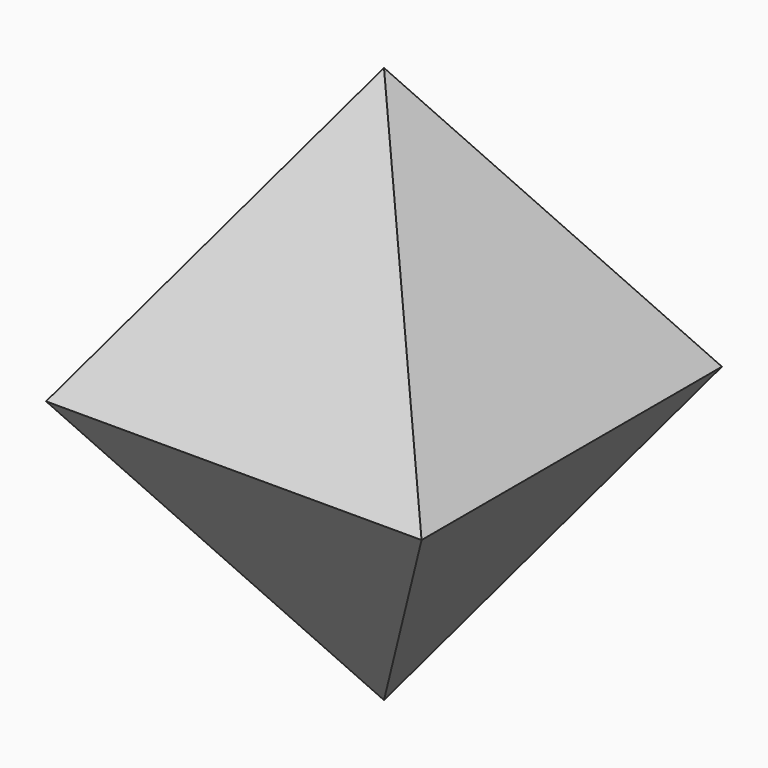
from build123d import *

# Parameters (mm, degrees)
F0_W      = 25.4
F0_H      = 25.4
F1_DEPTH  = 29.464
F1_TAPER  = 34
F1_FACE_W = 25.4
F1_FACE_H = 25.4


# Not quite as in the source:
# - an extrude whose draft closes it to a point is written as a loft to that point


with BuildPart() as f1:
    # F0 (on Top) → F1 (new body)
    with BuildSketch(Plane.XY):
        Rectangle(F0_W, F0_H)
    extrude(amount=F1_DEPTH, taper=F1_TAPER)

    # F1_face (on face) → F2 section 0
    with BuildSketch(Plane(origin=(0, 0, 0), x_dir=(1, 0, 0), z_dir=(0, 0, -1)), mode=Mode.PRIVATE) as f2_s0:
        Rectangle(F1_FACE_W, F1_FACE_H)
    loft([f2_s0.sketch, Vertex(0, 0, -18.8285243001)], ruled=True)


solid = f1.part
